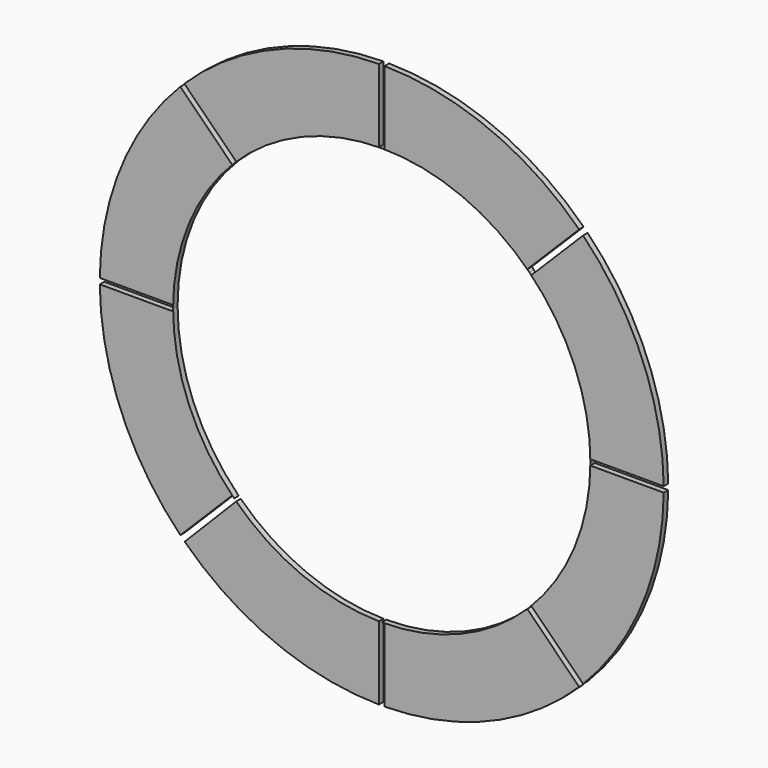
from build123d import *

# Parameters (mm, degrees)
F1_DEPTH = 6.35


with BuildPart() as f1:
    # F0 (on Front) → F1 (new body)
    with BuildSketch(Plane.XZ):
        with BuildLine():
            Line((234.95, -3.175), (234.95, 0))
            ThreePointArc((234.95, 0), (217.0654961635, -89.9114724342), (166.1347382398, -166.1347382398))
            Line((166.1347382398, -166.1347382398), (168.37980227, -163.8896742095))
            Line((168.37980227, -163.8896742095), (226.7402414562, -222.2501133957))
            ThreePointArc((226.7402414562, -222.2501133957), (293.3317515723, -121.5019897759), (317.4841246031, -3.175))
            Line((317.4841246031, -3.175), (234.95, -3.175))
        make_face()
    extrude(amount=F1_DEPTH)


with BuildPart() as f1b:
    # F0 (on Front) → F1, piece 2 (new body)
    with BuildSketch(Plane.XZ):
        with BuildLine():
            ThreePointArc((166.1347382398, 166.1347382398), (217.0654961635, 89.9114724342), (234.95, 0))
            Line((234.95, 0), (234.95, 3.175))
            Line((234.95, 3.175), (317.4841246031, 3.175))
            ThreePointArc((317.4841246031, 3.175), (293.3317515723, 121.5019897759), (226.7402414562, 222.2501133957))
            Line((226.7402414562, 222.2501133957), (168.37980227, 163.8896742095))
            Line((168.37980227, 163.8896742095), (166.1347382398, 166.1347382398))
        make_face()
    extrude(amount=F1_DEPTH)


with BuildPart() as f1c:
    # F0 (on Front) → F1, piece 3 (new body)
    with BuildSketch(Plane.XZ):
        with BuildLine():
            ThreePointArc((0, 234.95), (89.9114724342, 217.0654961635), (166.1347382398, 166.1347382398))
            Line((166.1347382398, 166.1347382398), (163.8896742095, 168.37980227))
            Line((163.8896742095, 168.37980227), (222.2501133957, 226.7402414562))
            ThreePointArc((222.2501133957, 226.7402414562), (121.5019897759, 293.3317515723), (3.175, 317.4841246031))
            Line((3.175, 317.4841246031), (3.175, 234.95))
            Line((3.175, 234.95), (0, 234.95))
        make_face()
    extrude(amount=F1_DEPTH)


with BuildPart() as f1d:
    # F0 (on Front) → F1, piece 4 (new body)
    with BuildSketch(Plane.XZ):
        with BuildLine():
            ThreePointArc((-166.1347382398, 166.1347382398), (-89.9114724342, 217.0654961635), (0, 234.95))
            Line((0, 234.95), (-3.175, 234.95))
            Line((-3.175, 234.95), (-3.175, 317.4841246031))
            ThreePointArc((-3.175, 317.4841246031), (-121.5019897759, 293.3317515723), (-222.2501133957, 226.7402414562))
            Line((-222.2501133957, 226.7402414562), (-163.8896742095, 168.37980227))
            Line((-163.8896742095, 168.37980227), (-166.1347382398, 166.1347382398))
        make_face()
    extrude(amount=F1_DEPTH)


with BuildPart() as f1e:
    # F0 (on Front) → F1, piece 5 (new body)
    with BuildSketch(Plane.XZ):
        with BuildLine():
            Line((222.2557078015, -226.7347577008), (163.8801180129, -168.3591679122))
            ThreePointArc((163.8801180129, -168.3591679122), (88.4463566209, -217.6665902257), (0, -234.95))
            Line((0, -234.95), (3.175, -234.95))
            Line((3.175, -234.95), (3.175, -317.4841246031))
            ThreePointArc((3.175, -317.4841246031), (121.505608526, -293.3302526108), (222.2557078015, -226.7347577008))
        make_face()
    extrude(amount=F1_DEPTH)


with BuildPart() as f1f:
    # F0 (on Front) → F1, piece 6 (new body)
    with BuildSketch(Plane.XZ):
        with BuildLine():
            ThreePointArc((-234.95, 0), (-217.0654961635, 89.9114724342), (-166.1347382398, 166.1347382398))
            Line((-166.1347382398, 166.1347382398), (-168.37980227, 163.8896742095))
            Line((-168.37980227, 163.8896742095), (-226.7402414562, 222.2501133957))
            ThreePointArc((-226.7402414562, 222.2501133957), (-293.3317515723, 121.5019897759), (-317.4841246031, 3.175))
            Line((-317.4841246031, 3.175), (-234.95, 3.175))
            Line((-234.95, 3.175), (-234.95, 0))
        make_face()
    extrude(amount=F1_DEPTH)


with BuildPart() as f1g:
    # F0 (on Front) → F1, piece 7 (new body)
    with BuildSketch(Plane.XZ):
        with BuildLine():
            ThreePointArc((-166.1347382398, -166.1347382398), (-217.0654961635, -89.9114724342), (-234.95, 0))
            Line((-234.95, 0), (-234.95, -3.175))
            Line((-234.95, -3.175), (-317.4841246031, -3.175))
            ThreePointArc((-317.4841246031, -3.175), (-293.3317515723, -121.5019897759), (-226.7402414562, -222.2501133957))
            Line((-226.7402414562, -222.2501133957), (-168.37980227, -163.8896742095))
            Line((-168.37980227, -163.8896742095), (-166.1347382398, -166.1347382398))
        make_face()
    extrude(amount=F1_DEPTH)


with BuildPart() as f1h:
    # F0 (on Front) → F1, piece 8 (new body)
    with BuildSketch(Plane.XZ):
        with BuildLine():
            Line((-3.1749275238, -317.4841253279), (-3.1749275238, -234.9285472973))
            ThreePointArc((-3.1749275238, -234.9285472973), (-89.9114724342, -217.0654961635), (-163.8745561064, -168.3645816701))
            Line((-163.8745561064, -168.3645816701), (-221.8514646433, -227.1303098127))
            ThreePointArc((-221.8514646433, -227.1303098127), (-121.2442670293, -293.4383712341), (-3.1749275238, -317.4841253279))
        make_face()
    extrude(amount=F1_DEPTH)


solid = Compound([f1.part, f1b.part, f1c.part, f1d.part, f1e.part, f1f.part, f1g.part, f1h.part])
